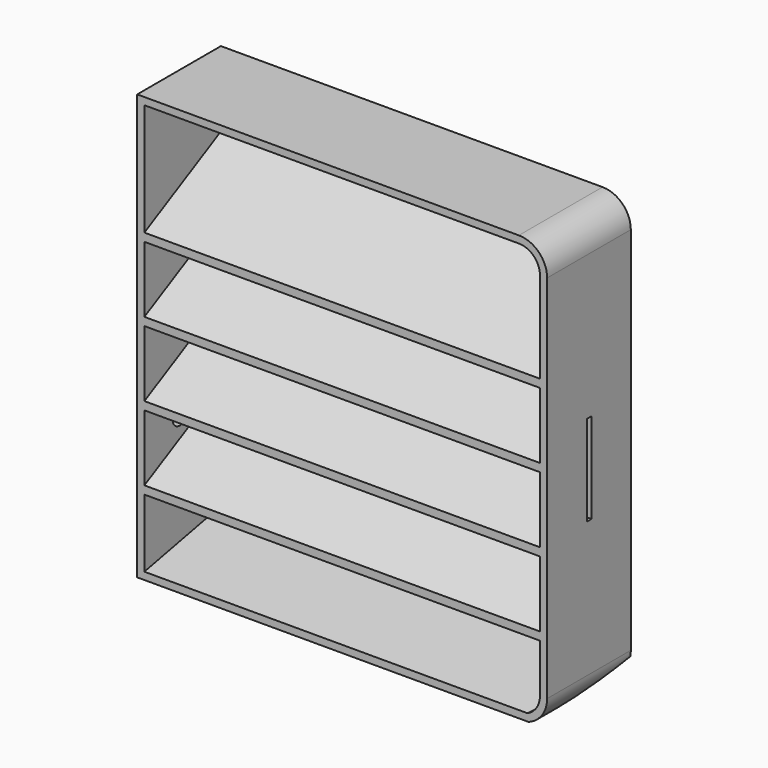
from build123d import *

# Parameters (mm, degrees)
F1_DEPTH    = 37
F2_T1_DEPTH = 342.8505669038
F3_T        = -2.54
F4_W        = 125.55387271
F4_H        = 111.9176980871
F5_DEPTH    = 25.4
F6_R        = 3.175
F7_DEPTH    = 19.05
F9_DEPTH    = 142.24
F10_W       = 2
F10_H       = 32
F11_DEPTH   = 5


# Not quite as in the source:
# - a fillet or chamfer that OpenCascade refuses, or shapes differently, is made with other operations: its cross-section is extruded or revolved along the edge and cut away or added


with BuildPart() as f1:
    # F0 (on Front) → F1 (new body)
    with BuildSketch(Plane.XZ):
        with BuildLine():
            Line((62.5, 75.5), (-72.5, 75.5))
            Line((-72.5, 75.5), (-72.5, -75.5))
            Line((-72.5, -75.5), (62.5, -75.5))
            ThreePointArc((62.5, -75.5), (69.5710678119, -72.5710678119), (72.5, -65.5))
            Line((72.5, -65.5), (72.5, 65.5))
            ThreePointArc((72.5, 65.5), (69.5710678119, 72.5710678119), (62.5, 75.5))
        make_face()
    extrude(amount=F1_DEPTH)

    # F2: chamfer of 40 x 8 on 1 edges, made by hand

    # F2_s2 → F2_t1 (cut)
    with BuildSketch(Plane.YZ.offset(-176.4252834519)):
        Polygon((-40, -75.5), (0, -67.5), (0, -75.5), align=None)
    extrude(amount=F2_T1_DEPTH, mode=Mode.SUBTRACT)

    # F3
    f3_openings = [f1.faces().sort_by_distance(p)[0] for p in [
        (-0.123954, -37, 0.284541),
    ]]
    offset(amount=F3_T, openings=f3_openings)

    # F4 (on face) → F5 (cut)
    with BuildSketch(Plane.XZ.offset(2.54)):
        with Locations((-0.276936355, 9.5411509565)):
            Rectangle(F4_W, F4_H)
    extrude(amount=-F5_DEPTH, mode=Mode.SUBTRACT)

    # F6 (on face) → F7 (cut)
    with BuildSketch(Plane(origin=(-72.5, 0, 0), x_dir=(0, -1, 0), z_dir=(-1, 0, 0))):
        with Locations((21.3561020792, 0)):
            Circle(F6_R)
        with Locations((21.3561020792, 35)):
            Circle(F6_R)
        with Locations((21.3561020792, -30)):
            Circle(F6_R)
    extrude(amount=-F7_DEPTH, mode=Mode.SUBTRACT)

    # F8 (on face) → F9 (join)
    with BuildSketch(Plane(origin=(69.96, 0, 0), x_dir=(0, -1, 0), z_dir=(-1, 0, 0))):
        Polygon((0, -28.8742875891), (37, -48.2893098931), (37, -45.4208615419), (0, -26.005839238), align=None)
        Polygon((0, -2.637839238), (37, -22.0528615419), (37, -19.1844131908), (0, 0.2306091132), align=None)
        Polygon((0, 23.5986091132), (37, 4.1835868092), (37, 7.0520351604), (0, 26.4670574643), align=None)
        Polygon((0, 49.8350574643), (37, 30.4200351604), (37, 33.2884835115), (0, 52.7035058155), align=None)
    extrude(amount=F9_DEPTH)

    # F10 (on face) → F11 (cut)
    with BuildSketch(Plane.YZ.offset(72.5)):
        with Locations((-18.3929149747, -1.5458973408)):
            Rectangle(F10_W, F10_H)
    extrude(amount=-F11_DEPTH, mode=Mode.SUBTRACT)


solid = f1.part
